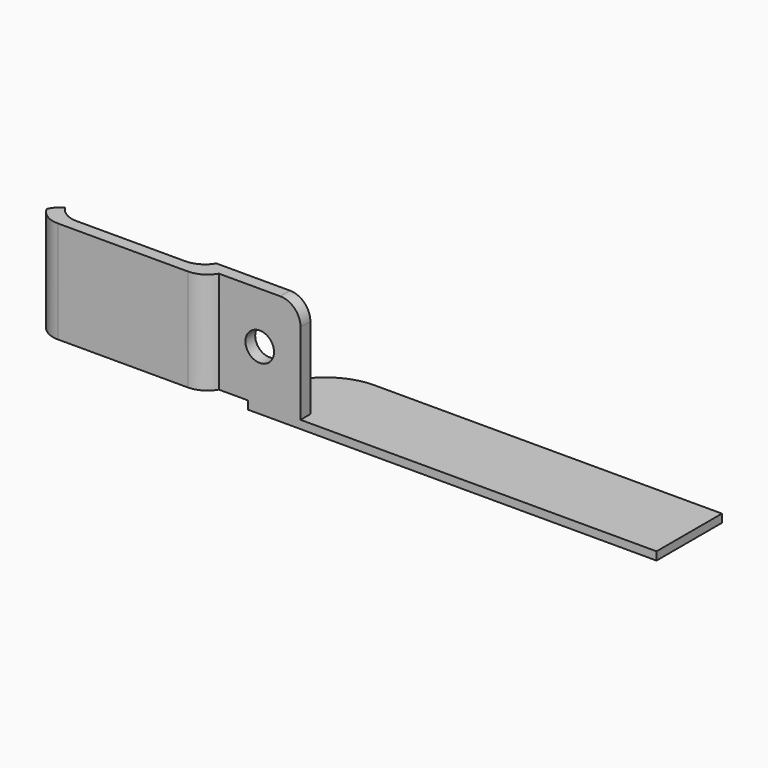
from build123d import *

# Parameters (mm, degrees)
F0_W        = 100
F0_H        = 20
F1_DEPTH    = 2
F2_R        = 15
F4_DEPTH    = 25
F5_T1_DEPTH = 25
F5_T3_DEPTH = 50.9807621135
F5_T5_DEPTH = 50.9793707428
F5_T7_DEPTH = 55
F6_R        = 5
F8_D        = 7


# Not quite as in the source:
# - a fillet or chamfer that OpenCascade refuses, or shapes differently, is made with other operations: its cross-section is extruded or revolved along the edge and cut away or added


with BuildPart() as f1:
    # F0 (on Top) → F1 (new body)
    with BuildSketch(Plane.XY):
        with Locations((46.6617465019, -62.7806016803)):
            Rectangle(F0_W, F0_H)
    extrude(amount=F1_DEPTH)

    # F2
    f2_edges = [f1.edges().sort_by_distance(p)[0] for p in [
        (-3.338253, -52.780602, 1),
    ]]
    fillet(f2_edges, radius=F2_R)

    # F3 (on face) → F4 (join)
    with BuildSketch(Plane.XY.offset(2)):
        Polygon((-10.4593388438, -72.7806016803), (9.5406611562, -72.7806016803), (9.5406611562, -69.7806016803), (-10.4593388438, -69.7806016803), (-13.4593388438, -69.7806016803), (-13.4593388438, -72.7806016803), (-50.4598207772, -72.7806016803), (-50.4598207772, -69.7806016803), (-53.4593388438, -69.7806016803), (-53.4593388438, -72.7806016803), (-53.4593388438, -75.7806016803), (-50.4598207772, -75.7806016803), (-13.4593388438, -75.7806016803), (-10.4593388438, -75.7806016803), align=None)
    extrude(amount=F4_DEPTH)

    # F5: fillet of radius 6 on 5 edges, made by hand

    # F5_s2 → F5_t1 (join)
    with BuildSketch(Plane.XY.offset(2)):
        with BuildLine():
            ThreePointArc((-13.4593388438, -69.7806016803), (-15.6554912665, -71.976754103), (-18.6554912665, -72.7806016803))
            Line((-18.6554912665, -72.7806016803), (-13.4593388438, -72.7806016803))
            Line((-13.4593388438, -72.7806016803), (-13.4593388438, -69.7806016803))
        make_face()
        with BuildLine():
            ThreePointArc((-50.4598207772, -69.7806016803), (-48.2636683545, -71.976754103), (-45.2636683545, -72.7806016803))
            Line((-45.2636683545, -72.7806016803), (-50.4598207772, -72.7806016803))
            Line((-50.4598207772, -72.7806016803), (-50.4598207772, -69.7806016803))
        make_face()
    extrude(amount=F5_T1_DEPTH)

    # F5_s4 → F5_t3 (cut)
    with BuildSketch(Plane.XY.offset(-10.9903810568)):
        with BuildLine():
            ThreePointArc((-10.4593388438, -72.7806016803), (-12.6554912665, -74.976754103), (-15.6554912665, -75.7806016803))
            Line((-15.6554912665, -75.7806016803), (-10.4593388438, -75.7806016803))
            Line((-10.4593388438, -75.7806016803), (-10.4593388438, -72.7806016803))
        make_face()
    extrude(amount=F5_T3_DEPTH, mode=Mode.SUBTRACT)

    # F5_s6 → F5_t5 (cut)
    with BuildSketch(Plane.XY.offset(-10.9896853714)):
        with BuildLine():
            ThreePointArc((-53.4593388438, -74.9764758288), (-52.6556303868, -71.9767168052), (-50.4598207772, -69.7806016803))
            Line((-50.4598207772, -69.7806016803), (-53.4593388438, -69.7806016803))
            Line((-53.4593388438, -69.7806016803), (-53.4593388438, -74.9764758288))
        make_face()
    extrude(amount=F5_T5_DEPTH, mode=Mode.SUBTRACT)

    # F5_s8 → F5_t7 (cut)
    with BuildSketch(Plane.XY.offset(-13)):
        with BuildLine():
            ThreePointArc((-47.4593388438, -75.7806016803), (-51.7019795309, -74.0232423674), (-53.4593388438, -69.7806016803))
            Line((-53.4593388438, -69.7806016803), (-53.4593388438, -75.7806016803))
            Line((-53.4593388438, -75.7806016803), (-47.4593388438, -75.7806016803))
        make_face()
    extrude(amount=F5_T7_DEPTH, mode=Mode.SUBTRACT)

    # F6
    f6_edges = [f1.edges().sort_by_distance(p)[0] for p in [
        (9.540661, -71.280602, 27),
    ]]
    fillet(f6_edges, radius=F6_R)

    # F8 (through all)
    with Locations(Plane.XZ.offset(72.7806016803)):
        with Locations((-0.4593388438, 14.5)):
            Hole(F8_D / 2)


solid = f1.part
